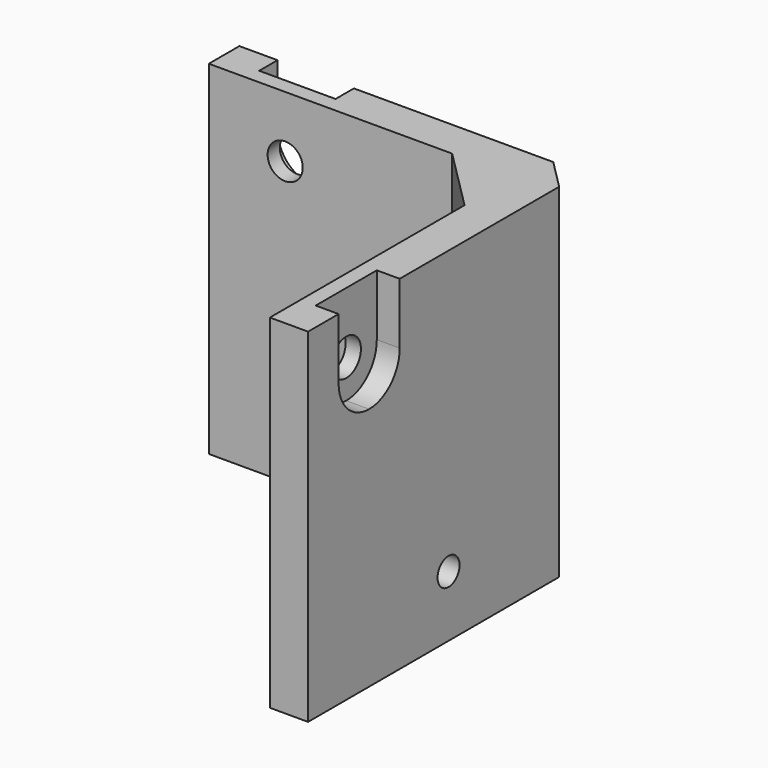
from build123d import *

# Parameters (mm, degrees)
F0_W      = 45
F0_H      = 45
F1_DEPTH  = 5
F2_W      = 45
F2_H      = 5
F3_DEPTH  = 40
F5_DEPTH  = 45
F7_DEPTH  = 45.001
F9_R      = 1.8
F9_R_2    = 2.3
F10_DEPTH = 45.001
F11_R     = 2.4
F11_R_2   = 1.8
F12_DEPTH = 45.001
F13_W     = 10
F13_H     = 3
F13_W_2   = 3
F13_H_2   = 10
F14_DEPTH = 13
F15_R     = 4.99999
F16_ANGLE = -90


# Not quite as in the source:
# - a fillet or chamfer is up to 0.001 mm smaller than in the source, because OpenCascade refuses the exact size


with BuildPart() as f1:
    # F0 (on Top) → F1 (new body)
    with BuildSketch(Plane.XY):
        Rectangle(F0_W, F0_H)
    extrude(amount=F1_DEPTH)

    # F2 (on face) → F3 (join)
    with BuildSketch(Plane.XY.offset(5)):
        with Locations((0, 20)):
            Rectangle(F2_W, F2_H)
    extrude(amount=F3_DEPTH)

    # F4 (on face) → F5 (join, through all)
    with BuildSketch(Plane(origin=(-22.5, 0, 0), x_dir=(0, -1, 0), z_dir=(-1, 0, 0))):
        Polygon((-9.3682720164, 5), (-17.5, 13.1317279836), (-17.5, 5), align=None)
    extrude(amount=-F5_DEPTH)

    # F6 (on face) → F7 (cut, through all)
    with BuildSketch(Plane.YZ.offset(22.5)):
        Polygon((18.6109127035, 0), (22.5, 0), (22.5, 3.8890872965), align=None)
    extrude(amount=-F7_DEPTH, mode=Mode.SUBTRACT)

    # F9 (on face) → F10 (cut, through all)
    with BuildSketch(Plane(origin=(0, 22.5, 0), x_dir=(-1, 0, 0), z_dir=(0, 1, 0))):
        with Locations((14.5, 22)):
            Circle(F9_R)
        with Locations((-14.5, 35)):
            Circle(F9_R_2)
    extrude(amount=-F10_DEPTH, mode=Mode.SUBTRACT)

    # F11 (on face) → F12 (cut, through all)
    with BuildSketch(Plane(origin=(0, 0, 0), x_dir=(1, 0, 0), z_dir=(0, 0, -1))):
        with Locations((14.5, 12.5)):
            Circle(F11_R)
        with Locations((-14.5, -0.5)):
            Circle(F11_R_2)
    extrude(amount=-F12_DEPTH, mode=Mode.SUBTRACT)

    # F13 (on face) → F14 (cut)
    with BuildSketch(Plane.YZ.offset(22.5)):
        with Locations((-12.5, 1.5)):
            Rectangle(F13_W, F13_H)
        with Locations((21, 35)):
            Rectangle(F13_W_2, F13_H_2)
    extrude(amount=-F14_DEPTH, mode=Mode.SUBTRACT)

    # F15 (radius 5 in the source; OpenCascade refuses exactly that, so slightly less here)
    f15_edges = [f1.edges().sort_by_distance(p)[0] for p in [
        (9.5, -17.5, 1.5),
        (9.5, -7.5, 1.5),
        (9.5, 21, 30),
        (9.5, 21, 40),
    ]]
    fillet(f15_edges, radius=F15_R)


with BuildPart() as f1_1:
    # F16: moved
    add(f1.part.rotate(Axis((-22.5, -1.9445436483, 0), (0, 1, 0)), F16_ANGLE))


with BuildPart() as f1_2:
    # F17: moved
    add(f1_1.part.moved(Location((40, 0, 0))))


solid = f1_2.part
